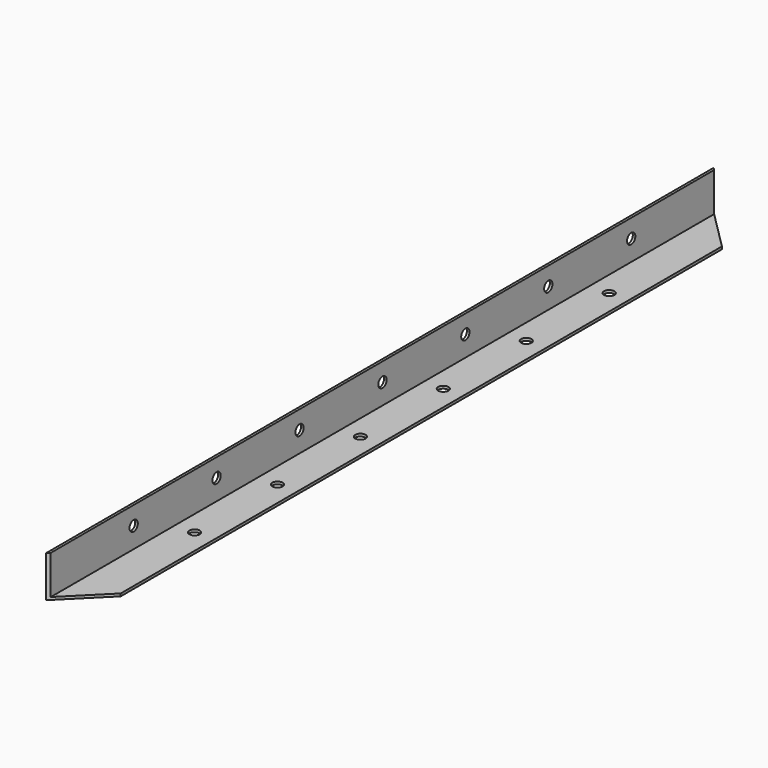
from build123d import *

# Parameters (mm, degrees)
F1_DEPTH = 1270
F3_DEPTH = 127
F5_DEPTH = 25.4
F6_R     = 6.35
F7_DEPTH = 25.4


# Not quite as in the source:
# - a feature names something its author has since deleted; it is built from what else it names


with BuildPart() as f1:
    # F0 (on Front) → F1 (new body)
    with BuildSketch(Plane.XZ):
        Polygon((3.175, 50.8), (0, 50.8), (0, 0), (50.8, 0), (50.8, 3.175), (3.175, 3.175), align=None)
    extrude(amount=F1_DEPTH)

    # F2 (on face) → F3 (intersect)
    with BuildSketch(Plane(origin=(0, 0, 0), x_dir=(1, 0, 0), z_dir=(0, 0, -1))):
        Polygon((0, 1022.35), (0, 0), (50.8, 50.8), (50.8, 971.55), align=None)
    extrude(amount=-F3_DEPTH, mode=Mode.INTERSECT)

    # F4 (on face) → F5 (cut)
    with BuildSketch(Plane.YZ.offset(3.175)):
        with BuildLine():
            ThreePointArc((-885.825155029, 28.3765627422), (-892.1701940961, 34.7265608044), (-898.5251472776, 28.3864846051))
            Line((-898.5251472776, 28.3864846051), (-885.8251627805, 28.3666408793))
            ThreePointArc((-885.8251627805, 28.3666408793), (-885.8251569669, 28.3716018093), (-885.825155029, 28.3765627422))
        make_face()
        with BuildLine():
            ThreePointArc((-123.825155029, 28.3765627422), (-130.7681849335, 34.6988104068), (-136.4143882675, 27.1956865442))
            Line((-136.4143882675, 27.1956865442), (-123.9396424845, 27.1761947539))
            ThreePointArc((-123.9396424845, 27.1761947539), (-123.8538416901, 27.7736550617), (-123.825155029, 28.3765627422))
        make_face()
        with BuildLine():
            Line((-123.9396424845, 27.1761947539), (-136.4143882675, 27.1956865442))
            ThreePointArc((-136.4143882675, 27.1956865442), (-130.1850768919, 22.0265704937), (-123.9396424845, 27.1761947539))
        make_face()
        with BuildLine():
            ThreePointArc((-250.825155029, 28.3765627422), (-257.6678327049, 34.7074211917), (-263.4487042283, 27.3941776629))
            Line((-263.4487042283, 27.3941776629), (-250.9047064081, 27.3745776663))
            ThreePointArc((-250.9047064081, 27.3745776663), (-250.8450741155, 27.8739937135), (-250.825155029, 28.3765627422))
        make_face()
        with BuildLine():
            Line((-250.9047064081, 27.3745776663), (-263.4487042283, 27.3941776629))
            ThreePointArc((-263.4487042283, 27.3941776629), (-257.1850768919, 22.0265704937), (-250.9047064081, 27.3745776663))
        make_face()
        with BuildLine():
            ThreePointArc((-377.825155029, 28.3765627422), (-384.567858719, 34.7144081026), (-390.4765830013, 27.5926587234))
            Line((-390.4765830013, 27.5926587234), (-377.8762075195, 27.5729706367))
            ThreePointArc((-377.8762075195, 27.5729706367), (-377.837931004, 27.9739566603), (-377.825155029, 28.3765627422))
        make_face()
        with BuildLine():
            Line((-377.8762075195, 27.5729706367), (-390.4765830013, 27.5926587234))
            ThreePointArc((-390.4765830013, 27.5926587234), (-384.1850768919, 22.0265704937), (-377.8762075195, 27.5729706367))
        make_face()
        with BuildLine():
            ThreePointArc((-504.825155029, 28.3765627422), (-511.4681836347, 34.7197980552), (-517.498110694, 27.7911298605))
            Line((-517.498110694, 27.7911298605), (-504.8540597111, 27.7713735308))
            ThreePointArc((-504.8540597111, 27.7713735308), (-504.8323853158, 28.0736232011), (-504.825155029, 28.3765627422))
        make_face()
        with BuildLine():
            Line((-504.8540597111, 27.7713735308), (-517.498110694, 27.7911298605))
            ThreePointArc((-517.498110694, 27.7911298605), (-511.1850768919, 22.0265704937), (-504.8540597111, 27.7713735308))
        make_face()
        with BuildLine():
            ThreePointArc((-631.825155029, 28.3765627422), (-638.3687307774, 34.7236115391), (-644.5133529596, 27.9895911765))
            Line((-644.5133529596, 27.9895911765), (-631.8381973298, 27.9697862458))
            ThreePointArc((-631.8381973298, 27.9697862458), (-631.8284164417, 28.1730699785), (-631.825155029, 28.3765627422))
        make_face()
        with BuildLine():
            Line((-631.8381973298, 27.9697862458), (-644.5133529596, 27.9895911765))
            ThreePointArc((-644.5133529596, 27.9895911765), (-638.1850768919, 22.0265704937), (-631.8381973298, 27.9697862458))
        make_face()
        with BuildLine():
            ThreePointArc((-758.825155029, 28.3765627422), (-765.2694254172, 34.7258629473), (-771.5223560035, 28.1880427438))
            Line((-771.5223560035, 28.1880427438), (-758.8285741702, 28.1682087096))
            ThreePointArc((-758.8285741702, 28.1682087096), (-758.8260098719, 28.2723716996), (-758.825155029, 28.3765627422))
        make_face()
        with BuildLine():
            Line((-758.8285741702, 28.1682087096), (-771.5223560035, 28.1880427438))
            ThreePointArc((-771.5223560035, 28.1880427438), (-765.1850768919, 22.0265704937), (-758.8285741702, 28.1682087096))
        make_face()
        with BuildLine():
            Line((-885.8251627805, 28.3666408793), (-898.5251472776, 28.3864846051))
            ThreePointArc((-898.5251472776, 28.3864846051), (-892.1850768919, 22.0265704937), (-885.8251627805, 28.3666408793))
        make_face()
    extrude(amount=-F5_DEPTH, mode=Mode.SUBTRACT)

    # F6 (on face) → F7 (cut)
    with BuildSketch(Plane.XY.offset(3.175)):
        with BuildLine():
            ThreePointArc((33.3375, -828.675), (22.4973719395, -824.1848719395), (26.9875, -835.025))
            ThreePointArc((26.9875, -835.025), (31.4776280605, -833.1651280605), (33.3375, -828.675))
        make_face()
        with Locations((26.9875, -701.675)):
            Circle(F6_R)
        with Locations((26.9875, -574.675)):
            Circle(F6_R)
        with Locations((26.9875, -447.675)):
            Circle(F6_R)
        with Locations((26.9875, -193.675)):
            Circle(F6_R)
        with Locations((26.9875, -320.675)):
            Circle(F6_R)
    extrude(amount=-F7_DEPTH, mode=Mode.SUBTRACT)


solid = f1.part
